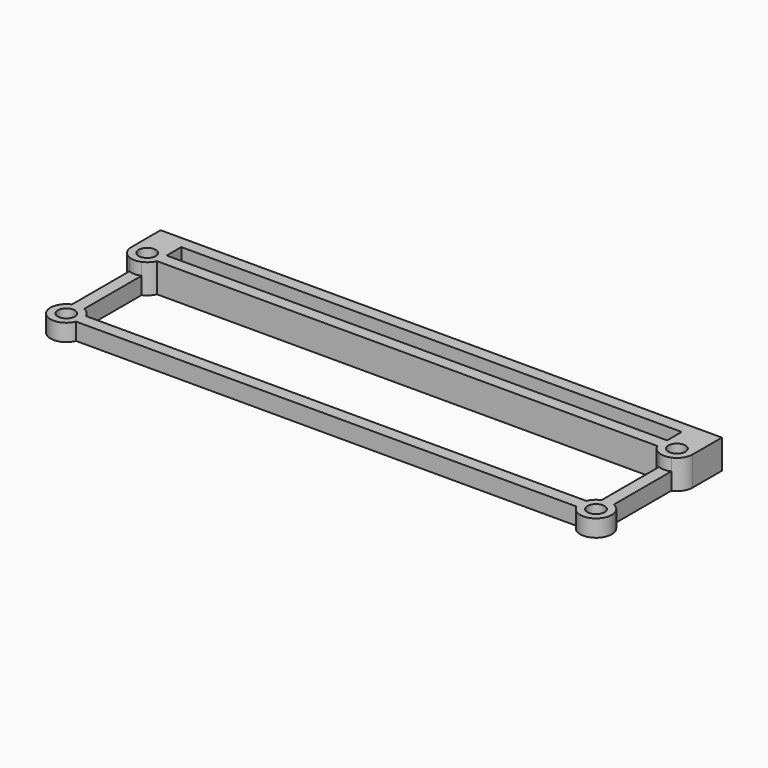
from build123d import *

# Parameters (mm, degrees)
F0_R     = 3.5
F0_W     = 205.5
F0_H     = 7.5
F1_DEPTH = 7
F2_R     = 3.5
F2_W     = 205.5
F2_H     = 7.5
F3_DEPTH = 5


# Not quite as in the source:
# - a feature of the source that left no trace in its solid (it failed there, or was rolled back) is left out


with BuildPart() as f1:
    # F0 (on Top) → F1 (new body)
    with BuildSketch(Plane.XY):
        with BuildLine():
            Line((-115.25, 43.0697486343), (-115.25, 28.0697486343))
            ThreePointArc((-115.25, 28.0697486343), (-114.1583269132, 24.4641973588), (-111.25, 22.0697486343))
            Line((-111.25, 22.0697486343), (-111.25, -7.4302513657))
            ThreePointArc((-111.25, -7.4302513657), (-113.3461940777, -18.0264454434), (-102.75, -15.9302513657))
            Line((-102.75, -15.9302513657), (102.75, -15.9302513657))
            ThreePointArc((102.75, -15.9302513657), (113.3461940777, -18.0264454434), (111.25, -7.4302513657))
            Line((111.25, -7.4302513657), (111.25, 22.0697486343))
            ThreePointArc((111.25, 22.0697486343), (114.1583269132, 24.4641973588), (115.25, 28.0697486343))
            Line((115.25, 28.0697486343), (115.25, 43.0697486343))
            Line((115.25, 43.0697486343), (-115.25, 43.0697486343))
        make_face()
        with Locations((-108.75, -13.4302513657)):
            Circle(F0_R, mode=Mode.SUBTRACT)
        with Locations((108.75, -13.4302513657)):
            Circle(F0_R, mode=Mode.SUBTRACT)
        with BuildLine():
            Line((-102.75, 25.5697486343), (102.75, 25.5697486343))
            ThreePointArc((102.75, 25.5697486343), (104.1538059223, 23.4735545566), (106.25, 22.0697486343))
            Line((106.25, 22.0697486343), (106.25, -7.4302513657))
            ThreePointArc((106.25, -7.4302513657), (104.1538059223, -8.834057288), (102.75, -10.9302513657))
            Line((102.75, -10.9302513657), (-102.75, -10.9302513657))
            ThreePointArc((-102.75, -10.9302513657), (-104.1538059223, -8.834057288), (-106.25, -7.4302513657))
            Line((-106.25, -7.4302513657), (-106.25, 22.0697486343))
            ThreePointArc((-106.25, 22.0697486343), (-104.1538059223, 23.4735545566), (-102.75, 25.5697486343))
        make_face(mode=Mode.SUBTRACT)
        with Locations((-108.75, 28.0697486343)):
            Circle(F0_R, mode=Mode.SUBTRACT)
        with Locations((0, 34.3197486343)):
            Rectangle(F0_W, F0_H, mode=Mode.SUBTRACT)
        with Locations((108.75, 28.0697486343)):
            Circle(F0_R, mode=Mode.SUBTRACT)
    extrude(amount=F1_DEPTH)

    # F2 (on face) → F3 (join)
    with BuildSketch(Plane.XY.offset(7)):
        with BuildLine():
            Line((115.25, 43.0697486343), (-115.25, 43.0697486343))
            Line((-115.25, 43.0697486343), (-115.25, 28.0697486343))
            ThreePointArc((-115.25, 28.0697486343), (-114.1583269132, 24.4641973588), (-111.25, 22.0697486343))
            ThreePointArc((-111.25, 22.0697486343), (-108.75, 21.5697486343), (-106.25, 22.0697486343))
            ThreePointArc((-106.25, 22.0697486343), (-104.1538059223, 23.4735545566), (-102.75, 25.5697486343))
            Line((-102.75, 25.5697486343), (102.75, 25.5697486343))
            ThreePointArc((102.75, 25.5697486343), (104.1538059223, 23.4735545566), (106.25, 22.0697486343))
            ThreePointArc((106.25, 22.0697486343), (108.75, 21.5697486343), (111.25, 22.0697486343))
            ThreePointArc((111.25, 22.0697486343), (114.1583269132, 24.4641973588), (115.25, 28.0697486343))
            Line((115.25, 28.0697486343), (115.25, 43.0697486343))
        make_face()
        with Locations((-108.75, 28.0697486343)):
            Circle(F2_R, mode=Mode.SUBTRACT)
        with Locations((108.75, 28.0697486343)):
            Circle(F2_R, mode=Mode.SUBTRACT)
        with Locations((0, 34.3197486343)):
            Rectangle(F2_W, F2_H, mode=Mode.SUBTRACT)
    extrude(amount=F3_DEPTH)


solid = f1.part
